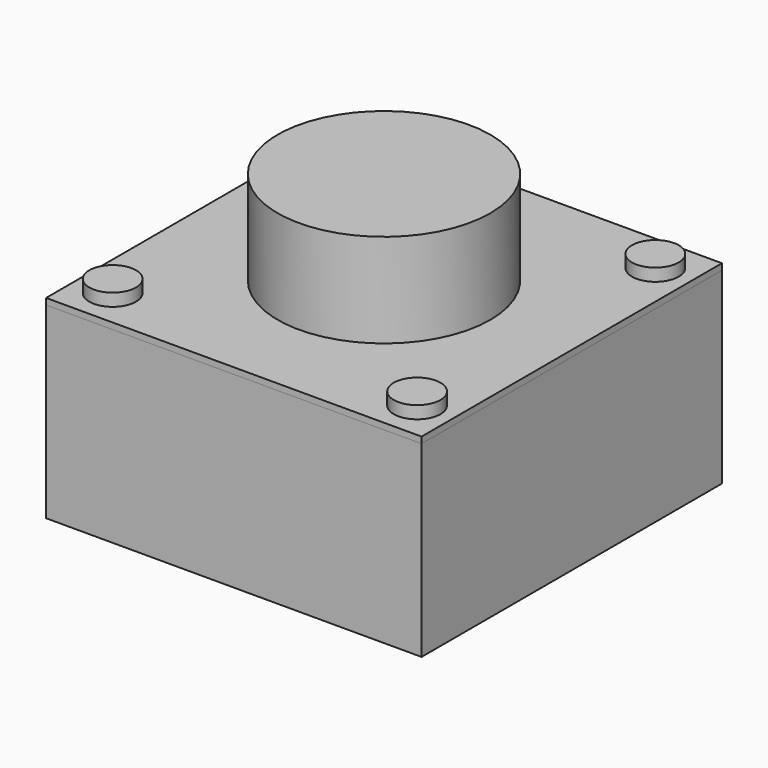
from build123d import *

# Parameters (mm, degrees)
F0_W     = 6
F0_H     = 6
F1_DEPTH = 3
F2_R     = 1.7
F3_DEPTH = 1.6
F4_DEPTH = 0.1
F2_R_2   = 0.3732558786
F5_DEPTH = 0.3


with BuildPart() as f1:
    # F0 (on Top) → F1 (new body)
    with BuildSketch(Plane.XY):
        Rectangle(F0_W, F0_H)
    extrude(amount=F1_DEPTH)


with BuildPart() as f3:
    # F2 (on face) → F3 (new body)
    with BuildSketch(Plane.XY.offset(3)):
        Circle(F2_R)
    extrude(amount=F3_DEPTH)


with BuildPart() as f4:
    # F4 (new): a face of the model
    f4_faces = [f1.part.faces().sort_by_distance(p)[0] for p in [
        (0, 0, 3),
    ]]
    extrude(f4_faces, amount=F4_DEPTH)


with BuildPart() as f1_1:
    add(f1.part)

    # F2 (on face) → F5 (join)
    with BuildSketch(Plane.XY.offset(3)):
        with Locations((-2.4326657876, -2.379177371)):
            Circle(F2_R_2)
        with Locations((2.4326657876, -2.379177371)):
            Circle(F2_R_2)
        with Locations((2.4326657876, 2.379177371)):
            Circle(F2_R_2)
        with Locations((-2.4326657876, 2.379177371)):
            Circle(F2_R_2)
    extrude(amount=F5_DEPTH)


solid = Compound([f3.part, f4.part, f1_1.part])
